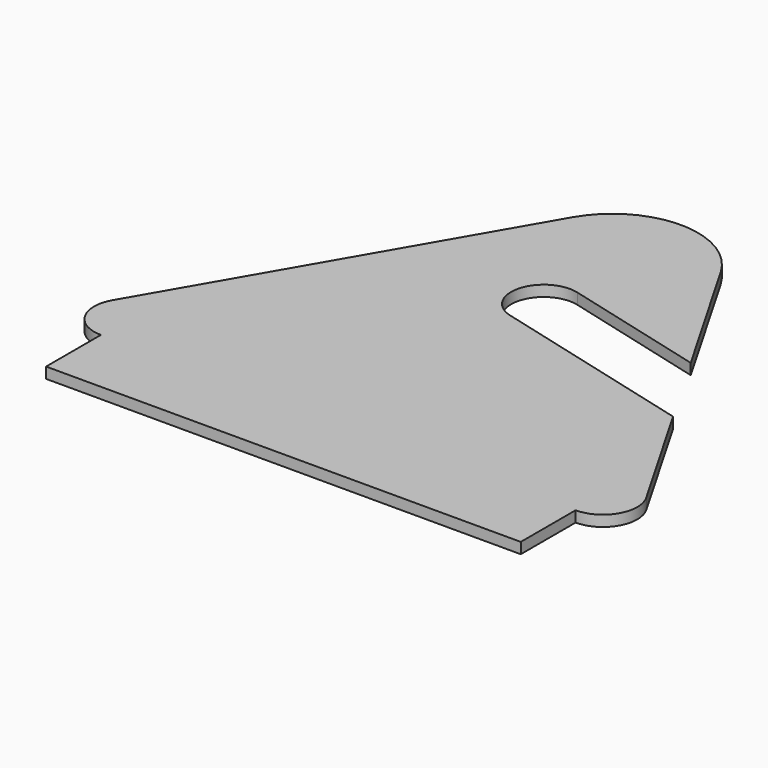
from build123d import *

# Parameters (mm, degrees)
F0_W     = 138.5640646055
F0_H     = 20
F1_DEPTH = 3.175
F3_DEPTH = 3.175


# Not quite as in the source:
# - a length typed as a fraction of an inch, garbled in the dataset ("3 / 203.2 mm" for 3/8 in), is restored


with BuildPart() as f1:
    # F0 (on Top) → F1 (new body)
    with BuildSketch(Plane.XY):
        with BuildLine():
            Line((77.9422863406, -35), (21.6506350946, 62.5))
            ThreePointArc((21.6506350946, 62.5), (0, 75), (-21.6506350946, 62.5))
            Line((-21.6506350946, 62.5), (-77.9422863406, -35))
            ThreePointArc((-77.9422863406, -35), (-77.9422863406, -45), (-69.2820323028, -50))
            Line((-69.2820323028, -50), (69.2820323028, -50))
            ThreePointArc((69.2820323028, -50), (77.9422863406, -45), (77.9422863406, -35))
        make_face()
        with Locations((0, -60)):
            Rectangle(F0_W, F0_H)
    extrude(amount=F1_DEPTH)

    # F2 (on face) → F3 (cut, through all)
    with BuildSketch(Plane.XY.offset(3.175)):
        with BuildLine():
            ThreePointArc((2.4179291552, 34.2129931944), (7.5417637262, 30.8178539771), (9.525, 25))
            ThreePointArc((9.525, 25), (5.8178542624, 17.4582364939), (-2.4179284582, 15.7870066226))
            Line((-2.4179284582, 15.7870066226), (57.735026919, 0))
            Line((57.735026919, 0), (44.3333494626, 23.2123862611))
            Line((44.3333494626, 23.2123862611), (2.4179291552, 34.2129931944))
        make_face()
        with BuildLine():
            ThreePointArc((-2.4179284582, 15.7870066226), (5.8178542624, 17.4582364939), (9.525, 25))
            ThreePointArc((9.525, 25), (7.5417637262, 30.8178539771), (2.4179291552, 34.2129931944))
            ThreePointArc((2.4179291552, 34.2129931944), (-9.2129932859, 27.4179288067), (-2.4179284582, 15.7870066226))
        make_face()
    extrude(amount=-F3_DEPTH, mode=Mode.SUBTRACT)


solid = f1.part
